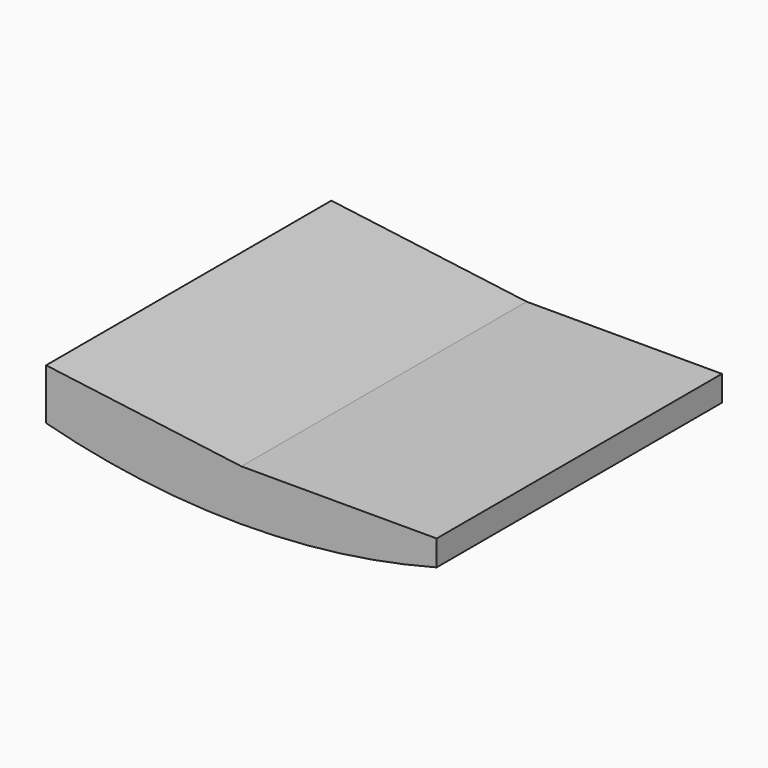
from build123d import *

# Parameters (mm, degrees)
F1_DEPTH = 420


# Not quite as in the source:
# - a feature names something its author has since deleted; it is built from what else it names


with BuildPart() as f1:
    # F0 (on Front) → F1 (new body)
    with BuildSketch(Plane.XZ):
        Polygon((-230, -30), (0, -30), (-230, 0), align=None)
        Polygon((0, -30), (230, -30), (230, 0), (0, 0), (-230, 30), (-230, 0), align=None)
        with BuildLine():
            ThreePointArc((-230, -30), (0, -60), (230, -30))
            Line((230, -30), (0, -30))
            Line((0, -30), (-230, -30))
        make_face()
    extrude(amount=-F1_DEPTH)


solid = f1.part
